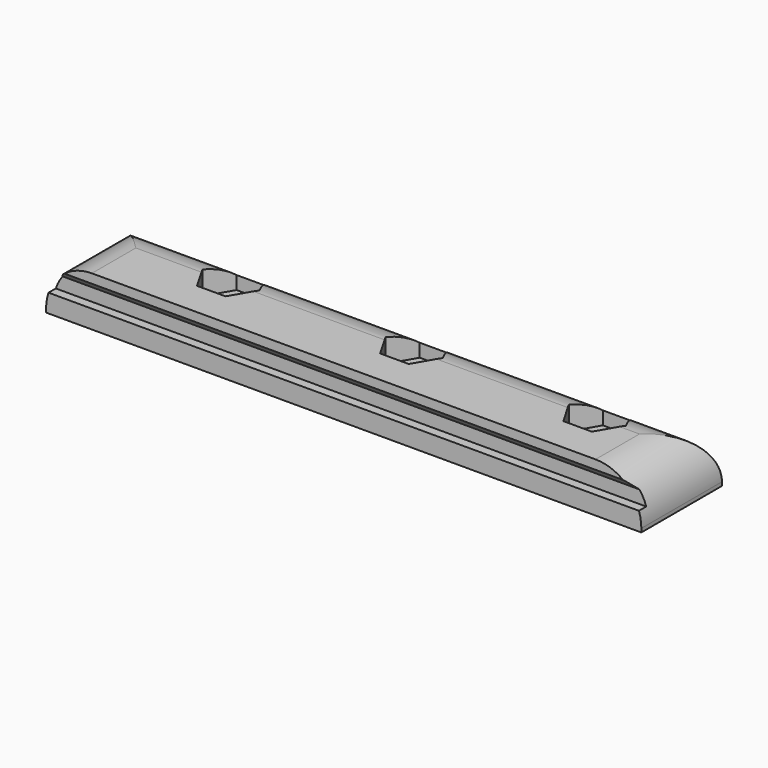
from build123d import *

# Parameters (mm, degrees)
F0_W        = 65
F0_H        = 5.4
F1_DEPTH    = 11
F2_W        = 65
F2_H        = 1.4
F3_DEPTH    = 1
F4_R        = 1.65
F5_DEPTH    = 25
F7_DEPTH    = 2.6
F8_T1_DEPTH = 36
F8_T3_DEPTH = 90
F9_SIZE     = 0.99999


# Not quite as in the source:
# - a fillet or chamfer that OpenCascade refuses, or shapes differently, is made with other operations: its cross-section is extruded or revolved along the edge and cut away or added
# - a fillet or chamfer is up to 0.001 mm smaller than in the source, because OpenCascade refuses the exact size


with BuildPart() as f1:
    # F0 (on Front) → F1 (new body)
    with BuildSketch(Plane.XZ):
        with Locations((32.1536201239, 16.5253020123)):
            Rectangle(F0_W, F0_H)
    extrude(amount=F1_DEPTH)

    # F2 (on face) → F3 (cut)
    with BuildSketch(Plane.XZ.offset(11)):
        with Locations((32.1536201239, 16.5253020123)):
            Rectangle(F2_W, F2_H)
    extrude(amount=-F3_DEPTH, mode=Mode.SUBTRACT)

    # F4 (on face) → F5 (cut)
    with BuildSketch(Plane.XY.offset(19.2253020123)):
        with Locations((14.6536201239, -4.5)):
            Circle(F4_R)
        with Locations((34.6536201239, -4.5)):
            Circle(F4_R)
        with Locations((54.6536201239, -4.5)):
            Circle(F4_R)
    extrude(amount=-F5_DEPTH, mode=Mode.SUBTRACT)

    # F6 (on face) → F7 (cut)
    with BuildSketch(Plane.XY.offset(19.2253020123)):
        Polygon((13.0947743971, -7.2), (16.2124658507, -7.2), (17.7713115775, -4.5), (16.2124658507, -1.8), (13.0947743971, -1.8), (11.5359286702, -4.5), align=None)
        Polygon((33.0947743971, -7.2), (36.2124658507, -7.2), (37.7713115775, -4.5), (36.2124658507, -1.8), (33.0947743971, -1.8), (31.5359286702, -4.5), align=None)
        Polygon((53.0947743971, -7.2), (56.2124658507, -7.2), (57.7713115775, -4.5), (56.2124658507, -1.8), (53.0947743971, -1.8), (51.5359286702, -4.5), align=None)
    extrude(amount=-F7_DEPTH, mode=Mode.SUBTRACT)

    # F8: fillet of radius 5 on 3 edges, made by hand

    # F8_s2 → F8_t1 (cut)
    with BuildSketch(Plane.XZ.offset(-12.5)):
        with BuildLine():
            ThreePointArc((64.6536201239, 14.2253020123), (63.1891540298, 17.7608359182), (59.6536201239, 19.2253020123))
            Line((59.6536201239, 19.2253020123), (64.6536201239, 19.2253020123))
            Line((64.6536201239, 19.2253020123), (64.6536201239, 14.2253020123))
        make_face()
        with BuildLine():
            ThreePointArc((4.6536201239, 19.2253020123), (1.1180862179, 17.7608359182), (-0.3463798761, 14.2253020123))
            Line((-0.3463798761, 14.2253020123), (-0.3463798761, 19.2253020123))
            Line((-0.3463798761, 19.2253020123), (4.6536201239, 19.2253020123))
        make_face()
    extrude(amount=F8_T1_DEPTH, mode=Mode.SUBTRACT)

    # F8_s4 → F8_t3 (cut)
    with BuildSketch(Plane.YZ.offset(-12.8463798761)):
        with BuildLine():
            ThreePointArc((0, 14.2253020123), (-1.4644660941, 17.7608359182), (-5, 19.2253020123))
            Line((-5, 19.2253020123), (0, 19.2253020123))
            Line((0, 19.2253020123), (0, 14.2253020123))
        make_face()
    extrude(amount=F8_T3_DEPTH, mode=Mode.SUBTRACT)

    # F9 (size 1 in the source; OpenCascade refuses exactly that, so slightly less here)
    f9_edges = [f1.edges().sort_by_distance(p)[0] for p in [
        (32.15362, -11, 17.225302),
    ]]
    chamfer(f9_edges, length=F9_SIZE)


solid = f1.part
